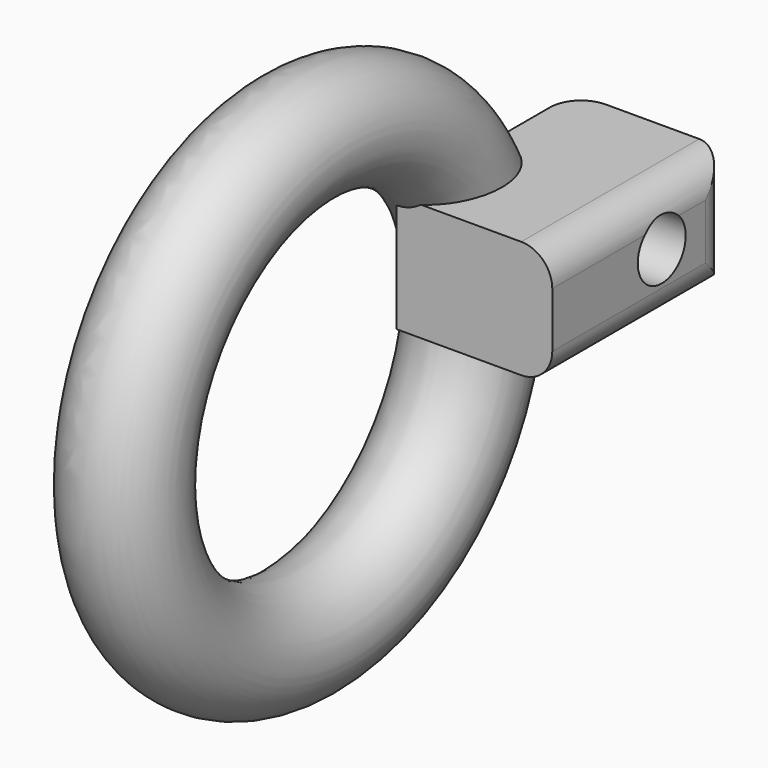
from build123d import *

# Parameters (mm, degrees)
F0_W        = 36.3452397287
F0_H        = 19.1822089255
F1_DEPTH    = 25.4
F2_R        = 4.8921614689
F3_DEPTH    = 25.4
F4_T1_DEPTH = 61.7452397287
F4_T3_DEPTH = 44.5822089255
F5_R        = 9.0132379352


# Not quite as in the source:
# - a fillet or chamfer that OpenCascade refuses, or shapes differently, is made with other operations: its cross-section is extruded or revolved along the edge and cut away or added


with BuildPart() as f1:
    # F0 (on Right) → F1 (new body)
    with BuildSketch(Plane.YZ):
        with Locations((18.1726198643, 9.5911044627)):
            Rectangle(F0_W, F0_H)
    extrude(amount=F1_DEPTH)

    # F2 (on face) → F3 (cut)
    with BuildSketch(Plane.YZ.offset(25.4)):
        with Locations((22.3394688219, 10.6473173946)):
            Circle(F2_R)
    extrude(amount=-F3_DEPTH, mode=Mode.SUBTRACT)

    # F4: fillet of radius 5.08 on 4 edges, made by hand

    # F4_s2 → F4_t1 (cut)
    with BuildSketch(Plane.XZ.offset(-49.0452397287)):
        with BuildLine():
            ThreePointArc((20.32, 0), (23.9121024484, 1.4878975516), (25.4, 5.08))
            Line((25.4, 5.08), (25.4, 0))
            Line((25.4, 0), (20.32, 0))
        make_face()
        with BuildLine():
            ThreePointArc((20.32, 19.1822089255), (23.9121024484, 17.6943113739), (25.4, 14.1022089255))
            Line((25.4, 14.1022089255), (25.4, 19.1822089255))
            Line((25.4, 19.1822089255), (20.32, 19.1822089255))
        make_face()
    extrude(amount=F4_T1_DEPTH, mode=Mode.SUBTRACT)

    # F4_s4 → F4_t3 (cut)
    with BuildSketch(Plane.XY.offset(-12.7)):
        with BuildLine():
            ThreePointArc((25.4, 31.2652397287), (23.9121024484, 34.8573421771), (20.32, 36.3452397287))
            Line((20.32, 36.3452397287), (25.4, 36.3452397287))
            Line((25.4, 36.3452397287), (25.4, 31.2652397287))
        make_face()
        with BuildLine():
            ThreePointArc((0, 31.2652397287), (1.4878975516, 34.8573421771), (5.08, 36.3452397287))
            Line((5.08, 36.3452397287), (0, 36.3452397287))
            Line((0, 36.3452397287), (0, 31.2652397287))
        make_face()
    extrude(amount=F4_T3_DEPTH, mode=Mode.SUBTRACT)

    # F5 (on Top) → F7 (revolve)
    with BuildSketch(Plane.XY):
        with Locations((0, -55.5648170412)):
            Circle(F5_R)
    revolve(axis=Axis((0, -19.9564255498, 0.2395265754), (1, 0, 0)))


solid = f1.part
